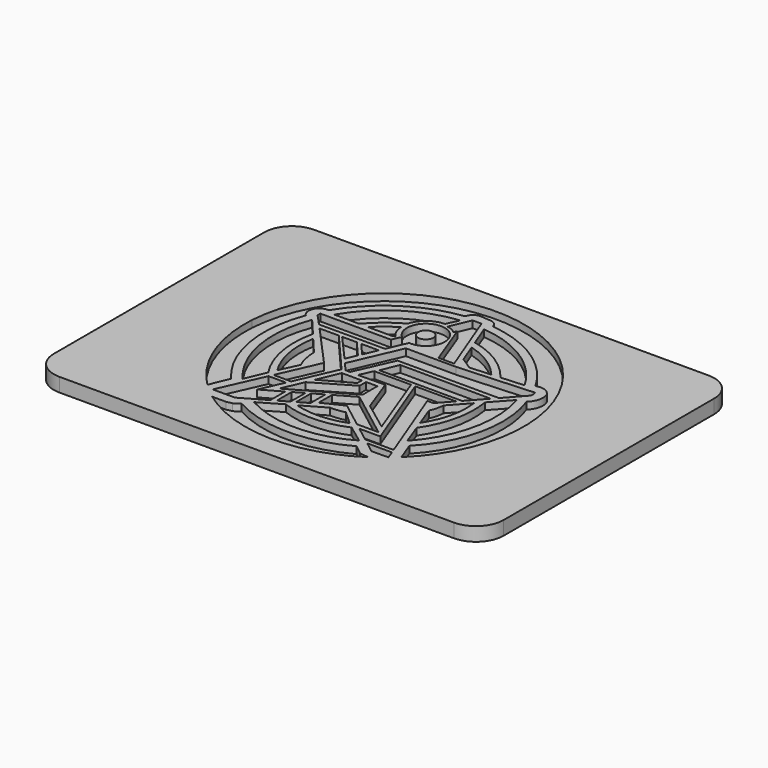
from build123d import *

# Parameters (mm, degrees)
F1_W     = 129.9656341411
F1_H     = 92
F2_DEPTH = 4
F0_R     = 2.206266784
F3_DEPTH = 2
F4_R     = 8


# Not quite as in the source:
# - a feature of the source that left no trace in its solid (it failed there, or was rolled back) is left out


with BuildPart() as f2:
    # F1 (on Top) → F2 (new body)
    with BuildSketch(Plane.XY):
        Rectangle(F1_W, F1_H)
    extrude(amount=-F2_DEPTH)

    # F0 (on Top) → F3 (cut)
    with BuildSketch(Plane.XY):
        with BuildLine():
            ThreePointArc((32.9198054021, 10.3452831455), (34.0598706525, -7.3543037213), (25.7183714124, -23.0066043337))
            Line((25.7183714124, -23.0066043337), (27.7859885246, -28.4340996295))
            ThreePointArc((27.7859885246, -28.4340996295), (40.0175359787, 1.9034119907), (25.6820959549, 31.3052915862))
            ThreePointArc((25.6820959549, 31.3052915862), (-16.0172109419, 37.1701752726), (-40.3886116997, 2.8297634895))
            ThreePointArc((-40.3886116997, 2.8297634895), (-37.7796921425, -13.9473169545), (-28.4849434409, -28.1559247702))
            Line((-28.4849434409, -28.1559247702), (-26.128076846, -22.5402322836))
            ThreePointArc((-26.128076846, -22.5402322836), (-34.0331337441, -6.0603942599), (-32.3028545506, 12.1352403748))
            ThreePointArc((-32.3028545506, 12.1352403748), (-32.9363949582, 15.6410225167), (-29.8190493924, 17.3655625997))
            ThreePointArc((-29.8190493924, 17.3655625997), (-18.8582022564, 28.8135157163), (-3.9804005212, 34.2767396752))
            ThreePointArc((-3.9804005212, 34.2767396752), (-3.0676094634, 35.7913755758), (-1.4240648597, 36.4441163838))
            Line((-1.4240648597, 36.4441163838), (2.2169065196, 36.2025946379))
            ThreePointArc((2.2169065196, 36.2025946379), (3.3586666016, 35.4777595975), (3.9804005212, 34.2767396752))
            ThreePointArc((3.9804005212, 34.2767396752), (18.8616664399, 29.0145635167), (29.7108907056, 17.5499699303))
            ThreePointArc((29.7108907056, 17.5499699303), (32.3169413343, 17.5683730236), (34.2922583222, 15.8683843911))
            ThreePointArc((34.2922583222, 15.8683843911), (34.4518228545, 12.896660486), (32.9198054021, 10.3452831455))
        make_face()
        with BuildLine():
            Line((-1.4240648597, 33.7512120605), (-3.9167157374, 27.8016738594))
            ThreePointArc((-3.9167157374, 27.8016738594), (-2.478492958, 27.411223522), (-1.2444847261, 26.5756638815))
            Line((-1.2444847261, 26.5756638815), (-0.7809350963, 27.4417696615))
            Line((-0.7809350963, 27.4417696615), (4.0169544055, 14.6583188688))
            Line((4.0169544055, 14.6583188688), (8.5247594051, 14.6583188688))
            Line((8.5247594051, 14.6583188688), (1.1711642146, 33.7512120605))
            Line((1.1711642146, 33.7512120605), (-1.4240648597, 33.7512120605))
        make_face()
        with BuildLine():
            Line((-8.1600512321, 10.558454176), (-5.7076071389, 16.1966606975))
            ThreePointArc((-5.7076071389, 16.1966606975), (-3.1111343426, 26.6870525684), (-8.7834731949, 17.4884350346))
            Line((-8.7834731949, 17.4884350346), (-9.9095003679, 14.8996813223))
            Line((-9.9095003679, 14.8996813223), (-30.3056854755, 14.8996813223))
            Line((-30.3056854755, 14.8996813223), (-30.3056854755, 13.8993896544))
            Line((-30.3056854755, 13.8993896544), (-27.2316206247, 10.558454176))
            Line((-27.2316206247, 10.558454176), (-8.1600512321, 10.558454176))
        make_face()
        with Locations((-5.2109998651, 21.5976983309)):
            Circle(F0_R, mode=Mode.SUBTRACT)
        with BuildLine():
            ThreePointArc((5.7671848814, 25.624841339), (14.2217691172, 22.0916254341), (20.9499727282, 15.8711041216))
            Line((20.9499727282, 15.8711041216), (27.5613053649, 16.3185875426))
            ThreePointArc((27.5613053649, 16.3185875426), (17.3583734285, 27.1277839963), (3.3137905526, 31.9948405928))
            Line((3.3137905526, 31.9948405928), (5.7671848814, 25.624841339))
        make_face()
        with BuildLine():
            ThreePointArc((8.9008489118, 17.4885881075), (10.6611040475, 16.477151656), (12.3050660696, 15.2859796666))
            Line((12.3050660696, 15.2859796666), (18.4604086408, 15.7025997193))
            ThreePointArc((18.4604086408, 15.7025997193), (13.1468531469, 20.4116151558), (6.6618675336, 23.301885033))
            Line((6.6618675336, 23.301885033), (8.9008489118, 17.4885881075))
        make_face()
        with BuildLine():
            ThreePointArc((-11.8280127645, 23.4212093055), (-9.3617553865, 27.0625318366), (-5.2014593966, 28.4885726869))
            Line((-5.2014593966, 28.4885726869), (-3.5191762727, 32.0172645152))
            ThreePointArc((-3.5191762727, 32.0172645152), (-17.3783821692, 27.0987516648), (-27.5436919183, 16.4716243744))
            Line((-27.5436919183, 16.4716243744), (-20.377356559, 16.4716243744))
            ThreePointArc((-20.377356559, 16.4716243744), (-16.4256839959, 20.3437689668), (-11.8280127645, 23.4212093055))
        make_face()
        with BuildLine():
            Line((-17.7911929276, 16.4569675014), (-10.7853559135, 16.4569675014))
            Line((-10.7853559135, 16.4569675014), (-10.1602249692, 16.7882594071))
            ThreePointArc((-10.1602249692, 16.7882594071), (-11.4433218227, 18.7755107075), (-11.9454109209, 21.0870928071))
            ThreePointArc((-11.9454109209, 21.0870928071), (-15.0373325891, 18.9854404517), (-17.7911929276, 16.4569675014))
        make_face()
        with BuildLine():
            Line((-8.5386522114, -3.1847900245), (-7.2461669333, -3.1847900245))
            Line((-7.2461669333, -3.1847900245), (-2.3474362679, 7.8362168339))
            Line((-2.3474362679, 7.8362168339), (26.9296697545, 7.8362168339))
            Line((26.9296697545, 7.8362168339), (31.6646508873, 13.1211960688))
            ThreePointArc((31.6646508873, 13.1211960688), (31.8589505472, 14.060598149), (31.5993018448, 14.9840759113))
            Line((31.5993018448, 14.9840759113), (9.8787359893, 13.6946468244))
            Line((9.8787359893, 13.6946468244), (-4.634531254, 13.6946468244))
            Line((-4.634531254, 13.6946468244), (-10.844227181, -0.5815391933))
            Line((-10.844227181, -0.5815391933), (-8.5386522114, -3.1847900245))
        make_face()
        Polygon((-8.7895971362, 9.1111185029), (-13.8198528439, 9.1111185029), (-10.5002270349, 5.178354173), align=None)
        Polygon((-15.1533698663, 9.1111185029), (-19.3795934319, 9.1111185029), (-12.2775910422, 1.0921671055), (-10.9149278039, 4.2249507552), align=None)
        Polygon((21.3057929504, 1.5590910554), (25.6767032032, 6.4377102676), (-0.5403367686, 6.5529635176), (-2.6323723141, 1.5590910554), align=None)
        Polygon((7.3953848332, 0.5306037302), (-3.2369155128, 0.5306037302), (-4.9318596721, -3.2547719311), (2.8672686312, -3.1235609204), (6.6189281642, -13.3572258055), (14.9748176336, -19.5951294154), align=None)
        Polygon((16.9147122651, -3.342041513), (20.384338416, 0.5306037302), (8.5737114516, 0.5306037302), (17.7439190447, -23.5232114792), (11.7003412661, -23.5232114792), (15.9513958452, -26.7689487949), (24.1976102576, -26.7689487949), (15.1895582676, -3.342041513), align=None)
        with BuildLine():
            ThreePointArc((25.7992849891, 4.2418451469), (25.5504244227, -5.8582983037), (21.5033187532, -15.1154990146))
            Line((21.5033187532, -15.1154990146), (23.82763608, -21.3668616892))
            ThreePointArc((23.82763608, -21.3668616892), (31.3748489247, -6.7863778514), (30.6619547671, 9.61614368))
            Line((30.6619547671, 9.61614368), (25.7992849891, 4.2418451469))
        make_face()
        with BuildLine():
            ThreePointArc((19.4215616787, -2.8069141965), (19.1068699093, -4.8492906233), (18.4095076227, -6.794545933))
            Line((18.4095076227, -6.794545933), (20.6188352743, -12.7366383735))
            ThreePointArc((20.6188352743, -12.7366383735), (23.7394905613, -5.4937999975), (24.1179729574, 2.3836328482))
            Line((24.1179729574, 2.3836328482), (19.4215616787, -2.8069141965))
        make_face()
        Polygon((-3.4139355139, -14.4867672903), (-3.4139355139, -19.3241007463), (2.4880508427, -16.4895039052), (9.9054172439, -22.1527628601), (16.1306671798, -22.1527628601), (2.0089598838, -11.384296231), align=None)
        Polygon((-8.3691851168, -4.7674076632), (-11.0682203042, -11.1124216708), (-2.5870061945, -6.3897371292), (-2.5870061945, -4.7674076632), align=None)
        Polygon((1.8993982812, -4.7674076632), (-1.3671386987, -4.7674076632), (-1.3671386987, -7.1084266528), (-12.0306818723, -13.3750198613), (-14.6343866363, -19.4959267974), (1.8993982812, -10.122532025), align=None)
        Polygon((-20.3438289464, 9.1111185029), (-25.8999802172, 9.1111185029), (-14.62478549, -3.3886153251), (-19.8245009044, -15.1117429357), (-14.757672244, -15.1117429357), (-9.5579568297, -3.3886153251), align=None)
        Polygon((-4.7273068426, -20.6174534154), (-4.7273068426, -15.2381549233), (-7.5725492149, -16.86593519), (-7.5725492149, -22.2452336821), align=None)
        with BuildLine():
            ThreePointArc((4.2871319637, -19.1493165641), (2.2119779448, -19.5473721372), (0.1005118497, -19.6275180716))
            Line((0.1005118497, -19.6275180716), (-6.4275181536, -23.3676129614))
            ThreePointArc((-6.4275181536, -23.3676129614), (0.990325371, -24.2978046546), (8.3078653292, -22.7670309614))
            Line((8.3078653292, -22.7670309614), (4.2871319637, -19.1493165641))
        make_face()
        with BuildLine():
            ThreePointArc((9.9917771295, -24.1659022868), (0.6767421733, -26.1995620096), (-8.7184906006, -24.5762169361))
            Line((-8.7184906006, -24.5762169361), (-14.9552477524, -28.228001669))
            ThreePointArc((-14.9552477524, -28.228001669), (0.1863431582, -32.1183821425), (15.2848139405, -28.0638765544))
            Line((15.2848139405, -28.0638765544), (9.9917771295, -24.1659022868))
        make_face()
        with BuildLine():
            Line((21.9549704343, -33.1265181303), (19.4017440081, -32.8504927456))
            Line((19.4017440081, -32.8504927456), (16.5863316506, -30.6085310876))
            ThreePointArc((16.5863316506, -30.6085310876), (-0.0233348713, -34.8399514885), (-16.6278406978, -30.5883251131))
            Line((-16.6278406978, -30.5883251131), (-18.358964473, -31.6868126392))
            Line((-18.358964473, -31.6868126392), (-20.0707614422, -32.0349745452))
            Line((-20.0707614422, -32.0349745452), (-24.0165982395, -32.0349745452))
            ThreePointArc((-24.0165982395, -32.0349745452), (-1.2023545282, -39.8053700313), (21.9549704343, -33.1265181303))
        make_face()
        with BuildLine():
            ThreePointArc((-18.0990044028, -7.4407774955), (-19.1800099478, -4.212385639), (-19.5703224259, -0.8302645387))
            Line((-19.5703224259, -0.8302645387), (-23.8585832759, 4.2575026946))
            ThreePointArc((-23.8585832759, 4.2575026946), (-23.846933184, -4.5646476853), (-20.5997571183, -12.7674716288))
            Line((-20.5997571183, -12.7674716288), (-18.0990044028, -7.4407774955))
        make_face()
        with BuildLine():
            ThreePointArc((-21.5105693248, -14.9086501639), (-25.62729083, -4.8126029101), (-25.4015651282, 6.0881591738))
            Line((-25.4015651282, 6.0881591738), (-29.8489369452, 11.3647021353))
            ThreePointArc((-29.8489369452, 11.3647021353), (-31.4735464013, -5.5945434485), (-24.077072315, -20.942101487))
            Line((-24.077072315, -20.942101487), (-21.5105693248, -14.9086501639))
        make_face()
        Polygon((-12.7012820409, -25.1794125656), (-12.7012820409, -19.8001140736), (-18.2435363531, -22.9708710854), (-15.2701737496, -16.2672139704), (-20.3445721418, -16.2672139704), (-26.118259877, -29.1949342936), (-19.7201240808, -29.1949342936), align=None)
        Polygon((-8.6919858711, -22.8856701231), (-8.6919858711, -17.5063716311), (-11.4179599798, -19.0659178071), (-11.4179599798, -24.4452162992), align=None)
        Polygon((24.6592686989, -27.96956681), (17.5238868432, -27.96956681), (20.7059439272, -30.3991101682), (25.5778580904, -30.3585082293), align=None)
    extrude(amount=-F3_DEPTH, mode=Mode.SUBTRACT)

    # F4
    f4_edges = [f2.edges().sort_by_distance(p)[0] for p in [
        (64.982817, 46, -2),
        (-64.982817, 46, -2),
        (-64.982817, -46, -2),
        (64.982817, -46, -2),
    ]]
    fillet(f4_edges, radius=F4_R)


solid = f2.part
